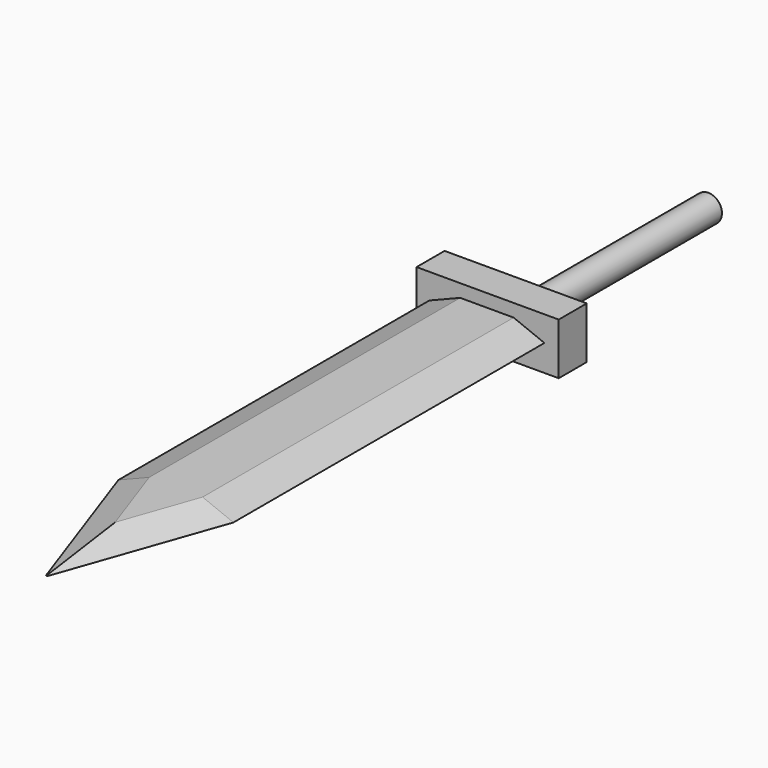
from build123d import *

# Parameters (mm, degrees)
F0_W        = 103.0951477587
F0_H        = 37.4727938324
F1_DEPTH    = 25.4
F2_R        = 9.8872931358
F3_DEPTH    = 165.1
F4_W        = 89.5363204181
F4_H        = 17.8772863001
F5_DEPTH    = 398.78
F6_T1_DEPTH = 464.6450864339
F7_SIZE2    = 116.84
F7_SIZE     = 15.24


# Not quite as in the source:
# - a fillet or chamfer that OpenCascade refuses, or shapes differently, is made with other operations: its cross-section is extruded or revolved along the edge and cut away or added


with BuildPart() as f1:
    # F0 (on Front) → F1 (new body)
    with BuildSketch(Plane.XZ):
        with Locations((-7.6333563775, 1.8935641274)):
            Rectangle(F0_W, F0_H)
    extrude(amount=F1_DEPTH)

    # F2 (on face) → F3 (join)
    with BuildSketch(Plane(origin=(0, 0, 0), x_dir=(-1, 0, 0), z_dir=(0, 1, 0))):
        Circle(F2_R)
    extrude(amount=F3_DEPTH)

    # F4 (on face) → F5 (join)
    with BuildSketch(Plane.XZ.offset(25.4)):
        with Locations((-8.1669483334, 2.3263469338)):
            Rectangle(F4_W, F4_H)
    extrude(amount=F5_DEPTH)

    # F6: chamfer of 25.4 x 10.16 on 4 edges, made by hand

    # F6_s2 → F6_t1 (cut)
    with BuildSketch(Plane.XZ.offset(25.4)):
        Polygon((-52.9351085424, 3.5477037838), (-27.5351085424, -6.6122962162), (-52.9351085424, -6.6122962162), align=None)
        Polygon((-27.5351085424, 11.2649900839), (-52.9351085424, 1.1049900839), (-52.9351085424, 11.2649900839), align=None)
        Polygon((11.2012118757, -6.6122962162), (36.6012118757, 3.5477037838), (36.6012118757, -6.6122962162), align=None)
        Polygon((11.2012118757, 11.2649900839), (36.6012118757, 1.1049900839), (36.6012118757, 11.2649900839), align=None)
    extrude(amount=F6_T1_DEPTH, mode=Mode.SUBTRACT)

    # F7 (call 1 of 2: OpenCascade refuses the feature's edges together)
    f7_edges = [f1.edges().sort_by_distance(p)[0] for p in [
        (-38.708412, -424.18, -2.142975),
        (-38.708412, -424.18, 6.795669),
    ]]
    f7_side = f1.faces().sort_by_distance((-8.166948, -424.18, 2.326347))[0]
    chamfer(f7_edges, length=F7_SIZE, length2=F7_SIZE2, reference=f7_side)

    # F7#2 (call 2 of 2)
    f7_2_edges = [f1.edges().sort_by_distance(p)[0] for p in [
        (22.374516, -424.18, -2.142975),
        (22.374516, -424.18, 6.795669),
    ]]
    f7_2_side = f1.faces().sort_by_distance((-8.166948, -424.18, 2.326347))[0]
    chamfer(f7_2_edges, length=F7_SIZE, length2=F7_SIZE2, reference=f7_2_side)


solid = f1.part
